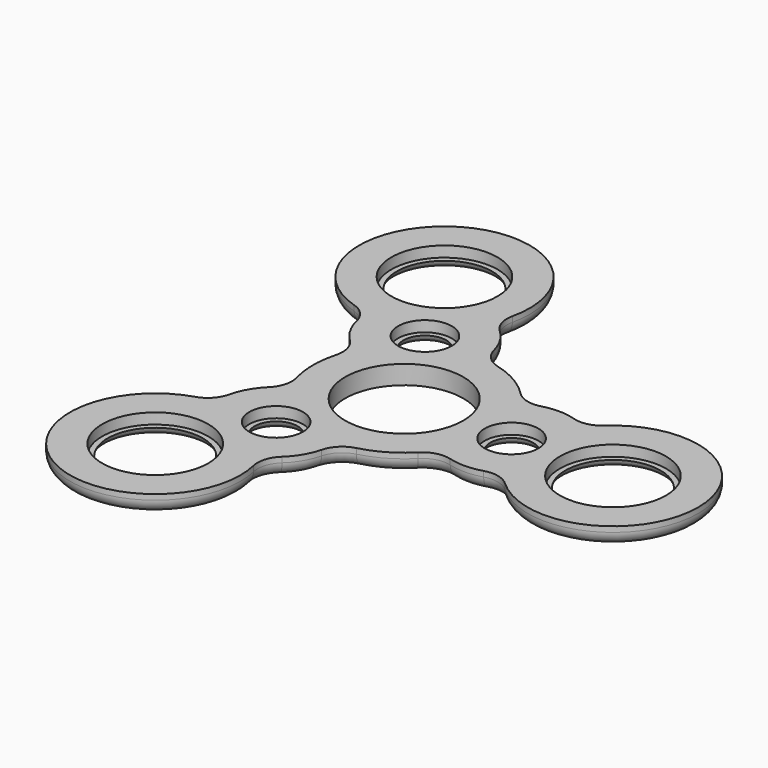
from build123d import *

# Parameters (mm, degrees)
F0_R     = 9.875
F0_R_2   = 5
F0_R_3   = 11
F1_DEPTH = 3.5
F0_R_4   = 8.875
F2_DEPTH = 1.5
F0_R_5   = 4
F3_DEPTH = 1.5
F4_R     = 2.5


# Not quite as in the source:
# - a fillet or chamfer that OpenCascade refuses, or shapes differently, is made with other operations: its cross-section is extruded or revolved along the edge and cut away or added


with BuildPart() as f1:
    # F0 (on Top) → F1 (new body)
    with BuildSketch(Plane.XY):
        with BuildLine():
            ThreePointArc((12.1318181818, -11.9087777544), (14.4083638811, -10.5810720707), (17.04375, -10.5953096197))
            ThreePointArc((17.04375, -10.5953096197), (20.1344758568, -10.9991779804), (23.2144039735, -10.5198672565))
            ThreePointArc((23.2144039735, -10.5198672565), (25.7947106614, -10.4284987853), (28.0765753262, -11.6365651961))
            ThreePointArc((28.0765753262, -11.6365651961), (54.75, 0), (28.0765753262, 11.6365651961))
            ThreePointArc((28.0765753262, 11.6365651961), (25.7947106614, 10.4284987853), (23.2144039735, 10.5198672565))
            ThreePointArc((23.2144039735, 10.5198672565), (20.1344758568, 10.9991779804), (17.04375, 10.5953096197))
            ThreePointArc((17.04375, 10.5953096197), (14.4083638811, 10.5810720707), (12.1318181818, 11.9087777544))
            ThreePointArc((12.1318181818, 11.9087777544), (8.5, 14.7224318643), (4.2473949724, 16.4608516167))
            ThreePointArc((4.2473949724, 16.4608516167), (1.9592952719, 17.7685451833), (0.6539322916, 20.0579752856))
            ThreePointArc((0.6539322916, 20.0579752856), (-0.5416703766, 22.936556574), (-2.4967296982, 25.364197203))
            ThreePointArc((-2.4967296982, 25.364197203), (-3.8660104593, 27.5531241087), (-3.9607265904, 30.1333100818))
            ThreePointArc((-3.9607265904, 30.1333100818), (-27.375, 47.4148908572), (-24.1158487357, 18.4967448857))
            ThreePointArc((-24.1158487357, 18.4967448857), (-21.9287002021, 17.1246253234), (-20.7176742754, 14.8443299465))
            ThreePointArc((-20.7176742754, 14.8443299465), (-19.5928054801, 11.9373785936), (-17.6976822916, 9.4626656659))
            ThreePointArc((-17.6976822916, 9.4626656659), (-16.367659153, 7.1874731127), (-16.3792131542, 4.5520738624))
            ThreePointArc((-16.3792131542, 4.5520738624), (-17, 0), (-16.3792131542, -4.5520738624))
            ThreePointArc((-16.3792131542, -4.5520738624), (-16.367659153, -7.1874731127), (-17.6976822916, -9.4626656659))
            ThreePointArc((-17.6976822916, -9.4626656659), (-19.5928054801, -11.9373785936), (-20.7176742754, -14.8443299465))
            ThreePointArc((-20.7176742754, -14.8443299465), (-21.9287002021, -17.1246253234), (-24.1158487357, -18.4967448857))
            ThreePointArc((-24.1158487357, -18.4967448857), (-27.375, -47.4148908572), (-3.9607265904, -30.1333100818))
            ThreePointArc((-3.9607265904, -30.1333100818), (-3.8660104593, -27.5531241087), (-2.4967296982, -25.364197203))
            ThreePointArc((-2.4967296982, -25.364197203), (-0.5416703766, -22.936556574), (0.6539322916, -20.0579752856))
            ThreePointArc((0.6539322916, -20.0579752856), (1.9592952719, -17.7685451833), (4.2473949724, -16.4608516167))
            ThreePointArc((4.2473949724, -16.4608516167), (8.5, -14.7224318643), (12.1318181818, -11.9087777544))
        make_face()
        with Locations((-19.4375, -33.6667375721)):
            Circle(F0_R, mode=Mode.SUBTRACT)
        with Locations((-10, -17.3205080757)):
            Circle(F0_R_2, mode=Mode.SUBTRACT)
        Circle(F0_R_3, mode=Mode.SUBTRACT)
        with Locations((-10, 17.3205080757)):
            Circle(F0_R_2, mode=Mode.SUBTRACT)
        with Locations((-19.4375, 33.6667375721)):
            Circle(F0_R, mode=Mode.SUBTRACT)
        with Locations((20, 0)):
            Circle(F0_R_2, mode=Mode.SUBTRACT)
        with Locations((38.875, 0)):
            Circle(F0_R, mode=Mode.SUBTRACT)
    extrude(amount=F1_DEPTH)

    # F0 (on Top) → F2 (join)
    with BuildSketch(Plane.XY):
        with Locations((-19.4375, 33.6667375721)):
            Circle(F0_R)
        with Locations((-19.4375, 33.6667375721)):
            Circle(F0_R_4, mode=Mode.SUBTRACT)
        with Locations((38.875, 0)):
            Circle(F0_R)
        with Locations((38.875, 0)):
            Circle(F0_R_4, mode=Mode.SUBTRACT)
        with Locations((-19.4375, -33.6667375721)):
            Circle(F0_R)
        with Locations((-19.4375, -33.6667375721)):
            Circle(F0_R_4, mode=Mode.SUBTRACT)
    extrude(amount=F2_DEPTH)

    # F0 (on Top) → F3 (join)
    with BuildSketch(Plane.XY):
        with Locations((20, 0)):
            Circle(F0_R_2)
        with Locations((20, 0)):
            Circle(F0_R_5, mode=Mode.SUBTRACT)
        with Locations((-10, -17.3205080757)):
            Circle(F0_R_2)
        with Locations((-10, -17.3205080757)):
            Circle(F0_R_5, mode=Mode.SUBTRACT)
        with Locations((-10, 17.3205080757)):
            Circle(F0_R_2)
        with Locations((-10, 17.3205080757)):
            Circle(F0_R_5, mode=Mode.SUBTRACT)
    extrude(amount=F3_DEPTH)

    # F4
    f4_edges = [f1.edges().sort_by_distance(p)[0] for p in [
        (-17, 0, 0),
        (-19.592805, 11.937379, 0),
        (-21.9287, 17.124625, 0),
        (-16.367659, 7.187473, 0),
        (-16.367659, -7.187473, 0),
        (-19.592805, -11.937379, 0),
        (-21.9287, -17.124625, 0),
        (-27.375, -47.414891, 0),
        (-3.86601, -27.553124, 0),
        (-0.54167, -22.936557, 0),
        (1.959295, -17.768545, 0),
        (8.5, -14.722432, 0),
        (14.408364, -10.581072, 0),
        (20.134476, -10.999178, 0),
        (25.794711, -10.428499, 0),
        (54.75, 0, 0),
        (25.794711, 10.428499, 0),
        (20.134476, 10.999178, 0),
        (14.408364, 10.581072, 0),
        (8.5, 14.722432, 0),
        (1.959295, 17.768545, 0),
        (-0.54167, 22.936557, 0),
        (-3.86601, 27.553124, 0),
        (-27.375, 47.414891, 0),
    ]]
    fillet(f4_edges, radius=F4_R)

    # F5: fillet of radius 2 on 6 edges, made by hand

    # F5_s1 → F5_t2 (revolve, cut)
    with BuildSketch(Plane.XZ.offset(-33.6667375721)):
        with BuildLine():
            ThreePointArc((-8.6260083269, 0), (-9.8507531983, 0.4188611699), (-10.5625, 1.5))
            Line((-10.5625, 1.5), (-10.5625, 0))
            Line((-10.5625, 0), (-8.6260083269, 0))
        make_face()
    revolve(axis=Axis((-19.4375, 33.6667375721, 0), (0, 0, 1)), mode=Mode.SUBTRACT)

    # F5_s3 → F5_t4 (revolve, cut)
    with BuildSketch(Plane.XZ.offset(-17.3205080757)):
        with BuildLine():
            ThreePointArc((-4.0635083269, 0), (-5.2882531983, 0.4188611699), (-6, 1.5))
            Line((-6, 1.5), (-6, 0))
            Line((-6, 0), (-4.0635083269, 0))
        make_face()
    revolve(axis=Axis((-10, 17.3205080757, 0), (0, 0, 1)), mode=Mode.SUBTRACT)

    # F5_s5 → F5_t6 (revolve, cut)
    with BuildSketch(Plane.XZ):
        with BuildLine():
            ThreePointArc((25.9364916731, 0), (24.7117468017, 0.4188611699), (24, 1.5))
            Line((24, 1.5), (24, 0))
            Line((24, 0), (25.9364916731, 0))
        make_face()
    revolve(axis=Axis((20, 0, 0), (0, 0, 1)), mode=Mode.SUBTRACT)

    # F5_s7 → F5_t8 (revolve, cut)
    with BuildSketch(Plane.XZ):
        with BuildLine():
            ThreePointArc((49.6864916731, 0), (48.4617468017, 0.4188611699), (47.75, 1.5))
            Line((47.75, 1.5), (47.75, 0))
            Line((47.75, 0), (49.6864916731, 0))
        make_face()
    revolve(axis=Axis((38.875, 0, 0), (0, 0, 1)), mode=Mode.SUBTRACT)

    # F5_s9 → F5_t10 (revolve, cut)
    with BuildSketch(Plane.XZ.offset(17.3205080757)):
        with BuildLine():
            ThreePointArc((-4.0635083269, 0), (-5.2882531983, 0.4188611699), (-6, 1.5))
            Line((-6, 1.5), (-6, 0))
            Line((-6, 0), (-4.0635083269, 0))
        make_face()
    revolve(axis=Axis((-10, -17.3205080757, 0), (0, 0, 1)), mode=Mode.SUBTRACT)

    # F5_s11 → F5_t12 (revolve, cut)
    with BuildSketch(Plane.XZ.offset(33.6667375721)):
        with BuildLine():
            ThreePointArc((-8.6260083269, 0), (-9.8507531983, 0.4188611699), (-10.5625, 1.5))
            Line((-10.5625, 1.5), (-10.5625, 0))
            Line((-10.5625, 0), (-8.6260083269, 0))
        make_face()
    revolve(axis=Axis((-19.4375, -33.6667375721, 0), (0, 0, 1)), mode=Mode.SUBTRACT)


solid = f1.part
